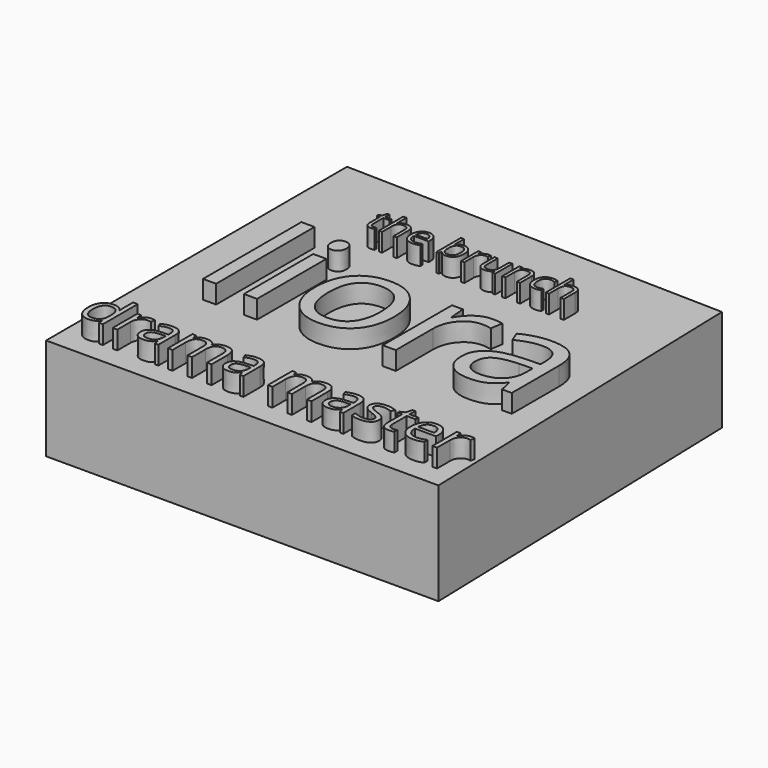
from build123d import *

# Parameters (mm, degrees)
F1_DEPTH     = 25.4
F4_TEXT_SIZE = 10.0038040222
F2_TEXT_SIZE = 40.3183577065
F3_TEXT_SIZE = 14.2478435818
F5_DEPTH     = 4.572


# Not quite as in the source:
# - Text() gives the source's letters only with a copy of the font that has no kerning and outlines rounded to 1/6400 em; it was checked with that copy


with BuildPart() as f1:
    # F0 (on Top) → F1 (new body)
    with BuildSketch(Plane.XY):
        Polygon((45.163795352, 43.8010953367), (-49.9656945467, 46.0073724389), (-49.9656945467, -47.6945266128), (47.7594174445, -47.6945266128), align=None)
    extrude(amount=F1_DEPTH)

    # F4 (on face) + F2 (on face) + F3 (on face) → F5 (join)
    with BuildSketch(Plane.XY.offset(25.4)):
        with Locations((-27.221522294, 21.9764709473)):
            Text('the brunch', F4_TEXT_SIZE, font='Open Sans', text_align=(TextAlign.LEFT, TextAlign.BOTTOM))
    with BuildSketch(Plane.XY.offset(25.4)):
        with Locations((-40.3172969818, -15.2376769111)):
            Text('liora', F2_TEXT_SIZE, font='Open Sans', text_align=(TextAlign.LEFT, TextAlign.BOTTOM))
    with BuildSketch(Plane.XY.offset(25.4)):
        with Locations((-47.6291663945, -42.3025116324)):
            Text('drama master', F3_TEXT_SIZE, font='Open Sans', text_align=(TextAlign.LEFT, TextAlign.BOTTOM))
    extrude(amount=F5_DEPTH)


solid = f1.part
